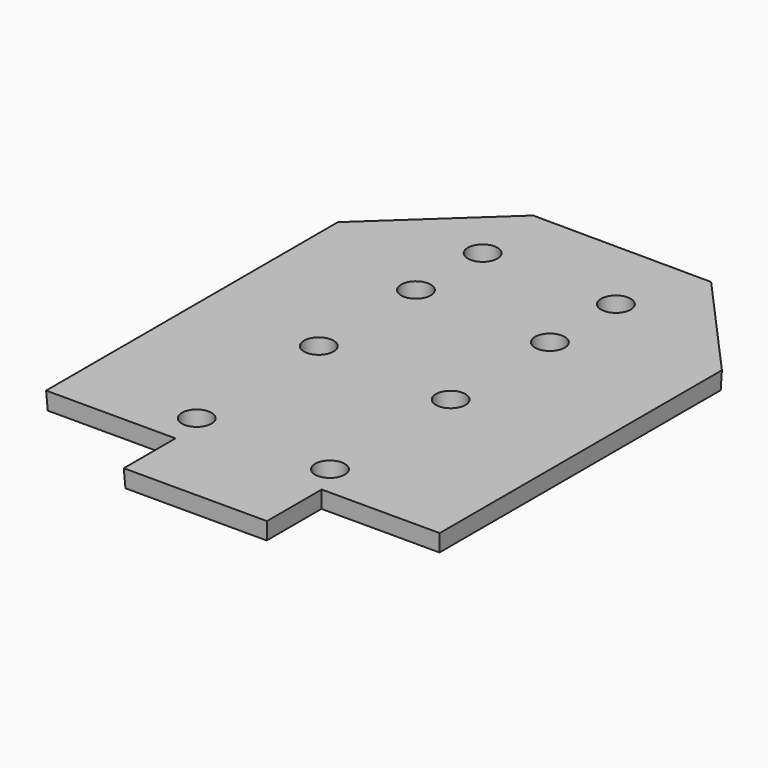
from build123d import *

# Parameters (mm, degrees)
F2_DEPTH   = 3
F2_TAPER   = -3
F6_D       = 5
F6_ON_F4_D = 5


# Not quite as in the source:
# - the program builds the solid bodies; features that only make, move or delete a surface that nothing else refers to are left out


with BuildPart() as f2:
    # F0 (on Top) → F2 (new body)
    with BuildSketch(Plane.XY):
        Polygon((-13.9245763421, -24.6634986252), (9.9384738132, -24.6634986252), (9.9384738132, -13.1047982723), (29.8719406128, -13.1047982723), (29.8719406128, 46.2553314865), (13.0966929719, 64.9538859725), (-16.9530268759, 65.1064962149), (-35.7809066772, 47.6274192333), (-35.7809066772, -13.7434657663), (-13.9245763421, -13.7434657663), align=None)
    extrude(amount=F2_DEPTH, taper=F2_TAPER)

    # F6 (through all)
    with Locations(Plane(origin=(0, 0, 0), x_dir=(1, 0, 0), z_dir=(0, 0, -1))):
        with Locations((-15.4966376722, -52.7129508555), (7.3292911984, -52.3064211011), (7.3292911984, -38.3762717247), (7.3292911984, -17.4282062799), (-15.4966376722, 7.6540475711), (7.3292911984, 8.0594113097)):
            Hole(F6_D / 2)

    # F6 on F4 (through all)
    with Locations(Plane(origin=(0, 0, 0), x_dir=(1, 0, 0), z_dir=(0, 0, -1))):
        with Locations((-15.7919153571, -38.9971844852), (-15.7919153571, -18.486443907)):
            Hole(F6_ON_F4_D / 2)


solid = f2.part
